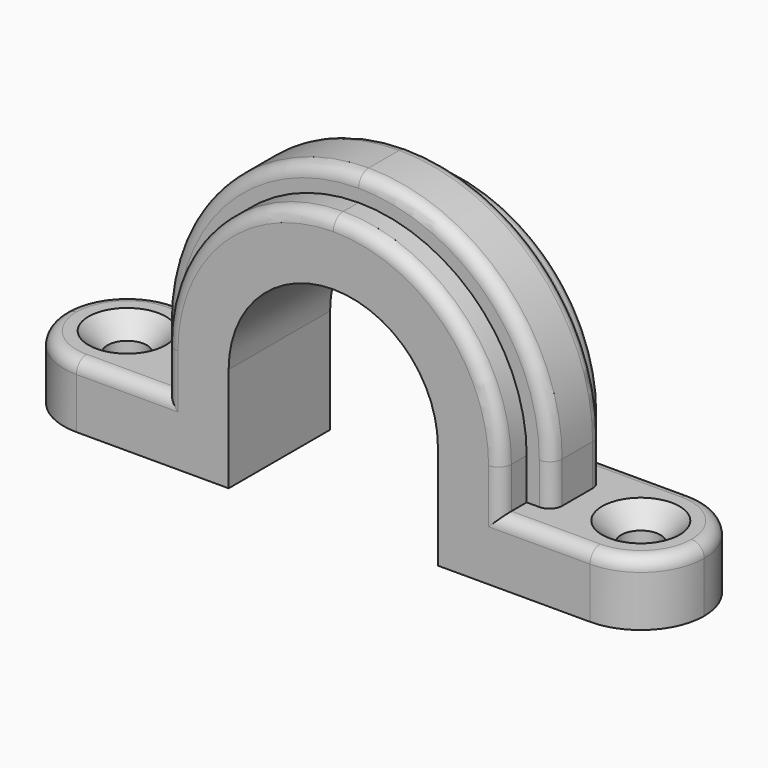
from build123d import *

# Parameters (mm, degrees)
F1_DEPTH        = 5
F2_DEPTH        = 2.5
F3_R            = 8.24999
F4_R            = 13.24999
F5_R            = 13.24999
F6_R            = 15.24999
F7_DEPTH        = 4
F8_DEPTH        = 4
F9_R            = 4.99999
F11_D           = 3.1
F11_CSINK_D     = 6.1
F11_CSINK_ANGLE = 90
F13_D           = 3.1
F13_CSINK_D     = 6.1
F13_CSINK_ANGLE = 90
F14_R           = 1


# Not quite as in the source:
# - a fillet or chamfer is up to 0.001 mm smaller than in the source, because OpenCascade refuses the exact size


with BuildPart() as f1:
    # F0 (on Front) → F1 (new body, symmetric)
    with BuildSketch(Plane.XZ):
        Polygon((-20.0976822525, 0), (-7.0976822525, 0), (-7.0976822525, 8.25), (-7.0976822525, 16.5), (9.4023177475, 16.5), (9.4023177475, 0), (22.4023177475, 0), (22.4023177475, 5), (16.4023177475, 5), (14.4023177475, 5), (14.4023177475, 21.5), (-12.0976822525, 21.5), (-12.0976822525, 5), (-14.0976822525, 5), (-20.0976822525, 5), align=None)
    extrude(amount=F1_DEPTH, both=True)

    # F0 (on Front) → F2 (join, symmetric)
    with BuildSketch(Plane.XZ):
        Polygon((-14.0976822525, 23.5), (-14.0976822525, 5), (-12.0976822525, 5), (-12.0976822525, 21.5), (14.4023177475, 21.5), (14.4023177475, 5), (16.4023177475, 5), (16.4023177475, 23.5), align=None)
    extrude(amount=F2_DEPTH, both=True)

    # F3 (radius 8.25 in the source; OpenCascade refuses exactly that, so slightly less here)
    f3_edges = [f1.edges().sort_by_distance(p)[0] for p in [
        (-7.097682, 0, 16.5),
        (9.402318, 0, 16.5),
    ]]
    fillet(f3_edges, radius=F3_R)

    # F4 (radius 13.25 in the source; OpenCascade refuses exactly that, so slightly less here)
    f4_edges = [f1.edges().sort_by_distance(p)[0] for p in [
        (14.402318, -3.75, 21.5),
        (-12.097682, -3.75, 21.5),
    ]]
    fillet(f4_edges, radius=F4_R)

    # F5 (radius 13.25 in the source; OpenCascade refuses exactly that, so slightly less here)
    f5_edges = [f1.edges().sort_by_distance(p)[0] for p in [
        (14.402318, 3.75, 21.5),
        (-12.097682, 3.75, 21.5),
    ]]
    fillet(f5_edges, radius=F5_R)

    # F6 (radius 15.25 in the source; OpenCascade refuses exactly that, so slightly less here)
    f6_edges = [f1.edges().sort_by_distance(p)[0] for p in [
        (16.402318, 0, 23.5),
        (-14.097682, 0, 23.5),
    ]]
    fillet(f6_edges, radius=F6_R)

    # F7 (add): a face of the model
    f7_faces = [f1.faces().sort_by_distance(p)[0] for p in [
        (22.4023177475, 0, 2.5),
    ]]
    extrude(f7_faces, amount=F7_DEPTH)

    # F8 (add): a face of the model
    f8_faces = [f1.faces().sort_by_distance(p)[0] for p in [
        (-20.0976822525, 0, 2.5),
    ]]
    extrude(f8_faces, amount=F8_DEPTH)

    # F9 (radius 5 in the source; OpenCascade refuses exactly that, so slightly less here)
    f9_edges = [f1.edges().sort_by_distance(p)[0] for p in [
        (26.402318, -5, 2.5),
        (26.402318, 5, 2.5),
        (-24.097682, -5, 2.5),
        (-24.097682, 5, 2.5),
    ]]
    fillet(f9_edges, radius=F9_R)

    # F11 (through all)
    with Locations(Plane.XY.offset(5)):
        with Locations((-19.0976822525, 0)):
            CounterSinkHole(F11_D / 2, F11_CSINK_D / 2, counter_sink_angle=F11_CSINK_ANGLE)

    # F13 (through all)
    with Locations(Plane.XY.offset(5)):
        with Locations((21.4023177475, 0)):
            CounterSinkHole(F13_D / 2, F13_CSINK_D / 2, counter_sink_angle=F13_CSINK_ANGLE)

    # F14
    f14_edges = [f1.edges().sort_by_distance(p)[0] for p in [
        (-9.631064, -2.5, 19.033381),
        (-9.631064, 2.5, 19.033381),
        (17.902323, 5, 5),
        (-15.597687, 5, 5),
        (-12.097682, 5, 6.625005),
        (-8.21685, 5, 17.619168),
        (1.152318, 5, 21.5),
        (10.521486, 5, 17.619168),
        (14.402318, 5, 6.625005),
        (-22.633219, 3.535537, 5),
        (-24.097682, 0, 5),
        (-22.633219, -3.535537, 5),
        (-15.597687, -5, 5),
        (17.902323, -5, 5),
        (24.937855, -3.535537, 5),
        (26.402318, 0, 5),
        (24.937855, 3.535537, 5),
        (-14.097682, 2.5, 6.625005),
        (1.152318, 2.5, 23.5),
        (11.935699, 2.5, 19.033381),
        (16.402318, 2.5, 6.625005),
        (-14.097682, -2.5, 6.625005),
        (-12.097682, -5, 6.625005),
        (-8.21685, -5, 17.619168),
        (1.152318, -5, 21.5),
        (10.521486, -5, 17.619168),
        (14.402318, -5, 6.625005),
        (1.152318, -2.5, 23.5),
        (11.935699, -2.5, 19.033381),
        (16.402318, -2.5, 6.625005),
    ]]
    fillet(f14_edges, radius=F14_R)


solid = f1.part
